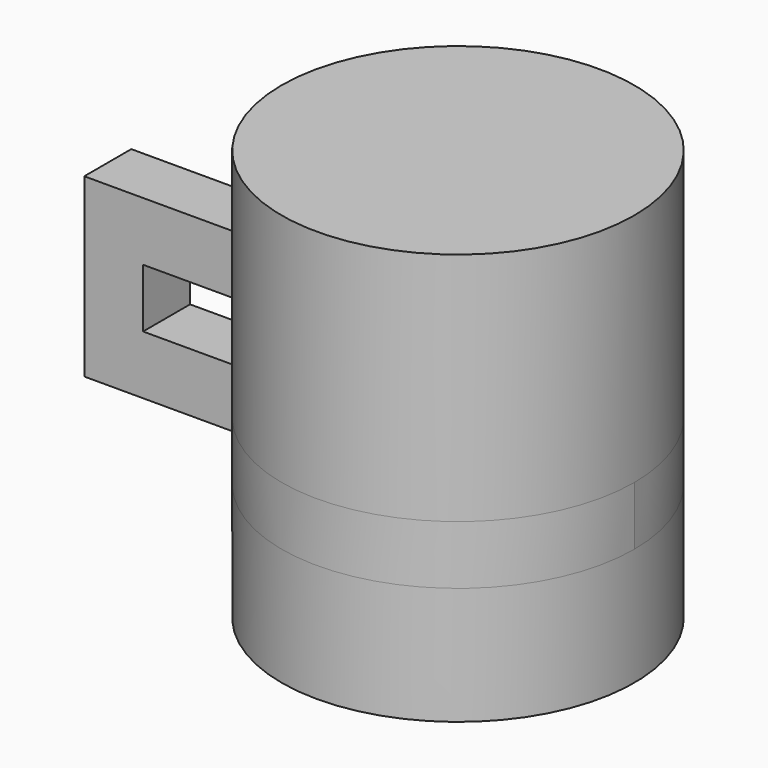
from build123d import *
from build123d import SkipClean  # not in build123d's __all__

# Parameters (mm, degrees)
F1_DEPTH      = 25.4
F2_R          = 76.2
F3_DEPTH      = 127
F4_DEPTH      = 50.8
F4_DEPTH_BACK = 25.4


with BuildPart() as f1:
    # F0 (on Front) → F1 (new body)
    with BuildSketch(Plane.XZ):
        Polygon((-12.3160492671, 73.0811166525), (-88.5160492671, 73.0811166525), (-88.5160492671, -3.1188833475), (-12.3160492671, -3.1188833475), (-12.3160492671, 22.2811166525), (-63.1160492671, 22.2811166525), (-63.1160492671, 47.6811166525), (-12.3160492671, 47.6811166525), align=None)
    extrude(amount=F1_DEPTH)

    # F2 (on Top) → F3 (join)
    with BuildSketch(Plane.XY):
        with Locations((62.8181639783, -12.7)):
            Circle(F2_R)
    extrude(amount=F3_DEPTH)

    # F4 (add, two sides): a face of the model
    f4_faces = [f1.faces().sort_by_distance(p)[0] for p in [
        (62.8930999906, -12.7, 0),
    ]]
    with SkipClean():  # cleaning this boolean's faces spoils the solid; the shape is the same uncleaned
        extrude(f4_faces, amount=F4_DEPTH)
        extrude(f4_faces, amount=-F4_DEPTH_BACK)


solid = f1.part
